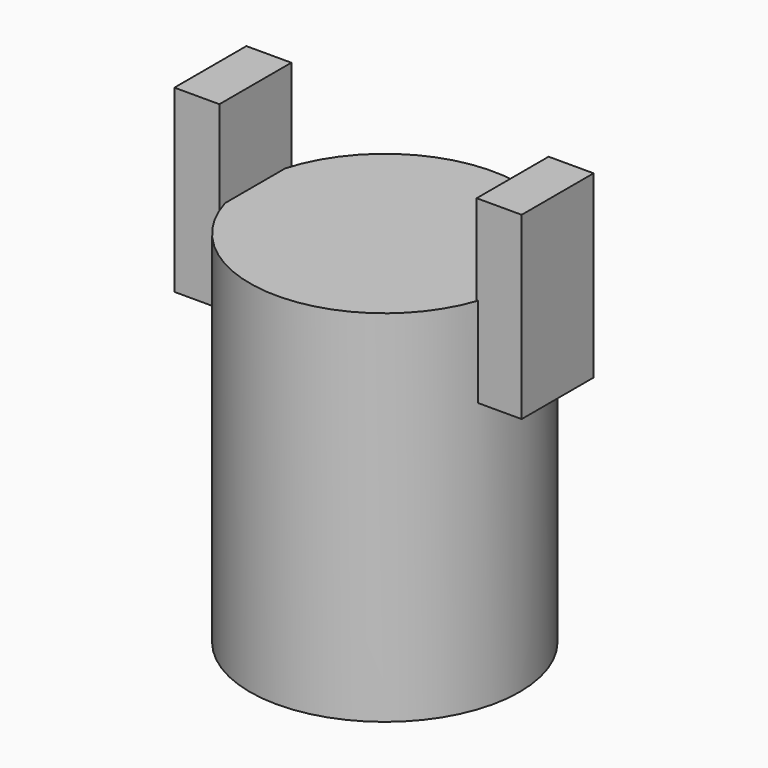
from build123d import *

# Parameters (mm, degrees)
F0_R     = 38.1
F1_DEPTH = 101.6
F2_W     = 12.7
F2_H     = 25.4
F3_DEPTH = 25.4


# Not quite as in the source:
# - a feature of the source that left no trace in its solid (it failed there, or was rolled back) is left out


with BuildPart() as f1:
    # F0 (on Top) → F1 (new body)
    with BuildSketch(Plane.XY):
        Circle(F0_R)
    extrude(amount=F1_DEPTH)

    # F2 (on face) → F3 (join, symmetric)
    with BuildSketch(Plane.XY.offset(101.6)):
        with Locations((-42.9418016334, 0.0489659142)):
            Rectangle(F2_W, F2_H)
        with Locations((42.1098351814, 0.4470220127)):
            Rectangle(F2_W, F2_H)
    extrude(amount=F3_DEPTH, both=True)


solid = f1.part
